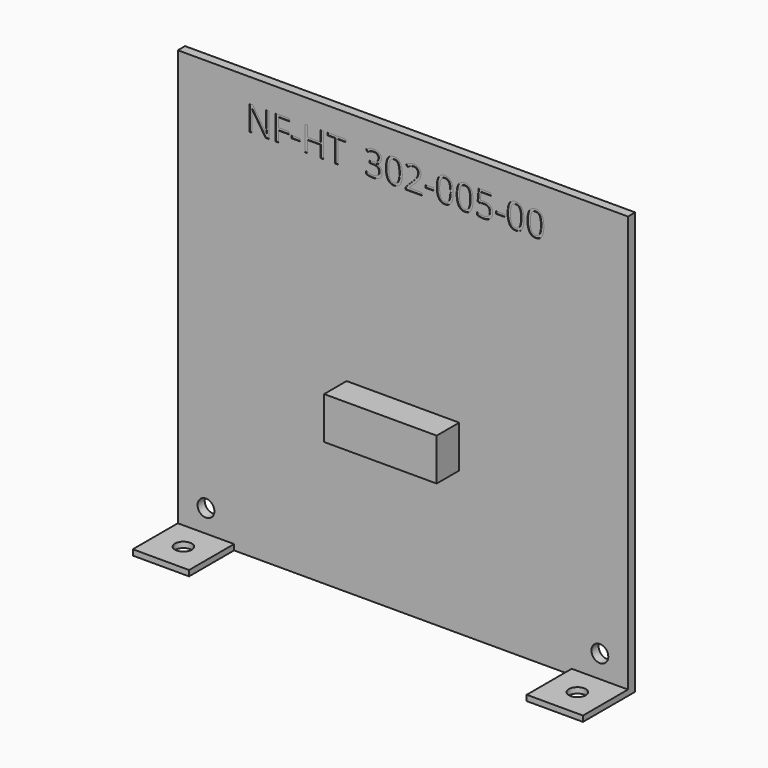
from build123d import *

# Parameters (mm, degrees)
F0_R         = 1.5
F0_W         = 20
F0_H         = 7.5
F0_W_2       = 10
F0_H_2       = 1
F1_DEPTH     = 1.6
F2_DEPTH     = 5
F3_TEXT_SIZE = 6.1743944469
F4_DEPTH     = 0.1
F5_DEPTH     = 10
F6_R         = 1.5
F7_DEPTH     = 1


# Not quite as in the source:
# - Text() gives the source's letters only with a copy of the font that has no kerning and outlines rounded to 1/6400 em; it was checked with that copy


with BuildPart() as f1:
    # F0 (on Front) → F1 (new body)
    with BuildSketch(Plane.XZ):
        Polygon((-30, -37.5), (30, -37.5), (30, -36.5), (40, -36.5), (40, 37.5), (-40, 37.5), (-40, -36.5), (-30, -36.5), align=None)
        with Locations((-35, -32.5)):
            Circle(F0_R, mode=Mode.SUBTRACT)
        with Locations((35, -32.5)):
            Circle(F0_R, mode=Mode.SUBTRACT)
        with Locations((0, -8.25)):
            Rectangle(F0_W, F0_H, mode=Mode.SUBTRACT)
        with Locations((0, -8.25)):
            Rectangle(F0_W, F0_H)
        with Locations((35, -37)):
            Rectangle(F0_W_2, F0_H_2)
        with Locations((-35, -37)):
            Rectangle(F0_W_2, F0_H_2)
    extrude(amount=-F1_DEPTH)

    # F0 (on Front) → F2 (join)
    with BuildSketch(Plane.XZ):
        with Locations((0, -8.25)):
            Rectangle(F0_W, F0_H)
    extrude(amount=F2_DEPTH)

    # F3 (on face) → F4 (cut)
    with BuildSketch(Plane.XZ):
        with Locations((-27.8697311878, 28.8684479892)):
            Text('NF-HT  302-005-00', F3_TEXT_SIZE, font='Open Sans', text_align=(TextAlign.LEFT, TextAlign.BOTTOM))
    extrude(amount=-F4_DEPTH, mode=Mode.SUBTRACT)

    # F0 (on Front) → F5 (join)
    with BuildSketch(Plane.XZ):
        with Locations((-35, -37)):
            Rectangle(F0_W_2, F0_H_2)
        with Locations((35, -37)):
            Rectangle(F0_W_2, F0_H_2)
    extrude(amount=F5_DEPTH)

    # F6 (on face) → F7 (cut, through all)
    with BuildSketch(Plane(origin=(0, 0, -37.5), x_dir=(1, 0, 0), z_dir=(0, 0, -1))):
        with Locations((-35, 5)):
            Circle(F6_R)
        with Locations((35, 5)):
            Circle(F6_R)
    extrude(amount=-F7_DEPTH, mode=Mode.SUBTRACT)


solid = f1.part
